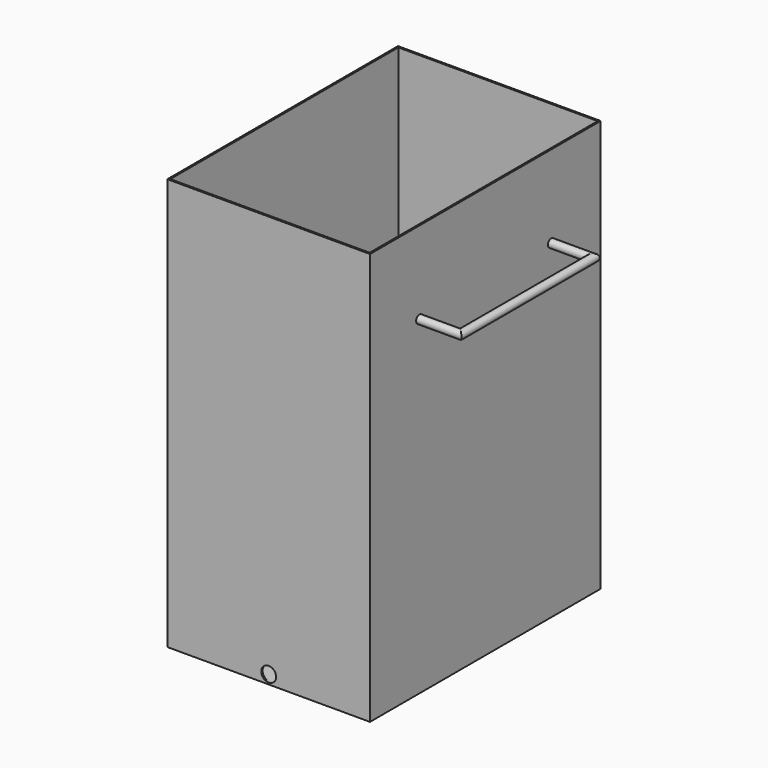
from build123d import *

# Parameters (mm, degrees)
F1_DEPTH  = 123
F4_DEPTH  = 2
F12_DEPTH = 500


# Not quite as in the source:
# - a feature names something its author has since deleted; it is built from what else it names


with BuildPart() as f1:
    # F0 (on Right) → F1 (new body)
    with BuildSketch(Plane.YZ):
        Polygon((175, -500), (175, 0), (173, 0), (173, -498), (-173, -498), (-173, 0), (-175, 0), (-175, -500), align=None)
    extrude(amount=F1_DEPTH)

    # F3 (on offset) → F4 (join)
    with BuildSketch(Plane.YZ.offset(123)):
        Polygon((175, 0), (0, 0), (-175, 0), (-175, -500), (175, -500), align=None)
    extrude(amount=-F4_DEPTH)

    # F9: F1, F8 across face


with BuildPart() as f8:
    # F8: sweep along a path in F7
    with BuildLine(Plane.XY.offset(-100)) as f8_path:
        Line((123, 100), (173, 100))
        Line((173, 100), (173, -100))
        Line((173, -100), (123, -100))
    # F5 (on offset) → F8 (sweep)
    with BuildSketch(Plane.YZ.offset(123)):
        with BuildLine():
            ThreePointArc((95, -100), (100, -105), (105, -100))
            ThreePointArc((105, -100), (100, -95), (95, -100))
        make_face()
    sweep(path=f8_path.line, transition=Transition.RIGHT)


with BuildPart() as f1_1:
    add(f1.part)
    add(f1.part.mirror(Plane(origin=(0, 0, -314.0074294205), x_dir=(0, 1, 0), z_dir=(-1, 0, 0))))
    add(f8.part.mirror(Plane(origin=(0, 0, -314.0074294205), x_dir=(0, 1, 0), z_dir=(-1, 0, 0))))

    # F11 (on offset) → F12 (cut)
    with BuildSketch(Plane.XZ.offset(175)):
        with BuildLine():
            ThreePointArc((0, -480), (-6.3639610307, -495.3639610307), (9, -489))
            ThreePointArc((9, -489), (6.3639610307, -482.6360389693), (0, -480))
        make_face()
    extrude(amount=-F12_DEPTH, mode=Mode.SUBTRACT)


solid = Compound([f8.part, f1_1.part])
